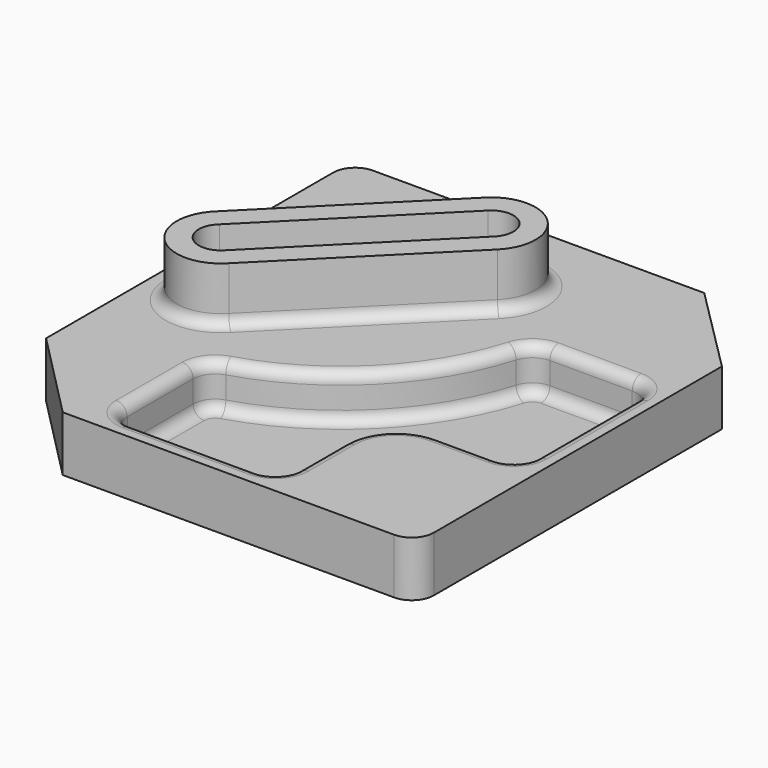
from build123d import *

# Parameters (mm, degrees)
F1_DEPTH = 25
F4_DEPTH = 25
F5_DEPTH = 5
F6_R     = 5
F7_R     = 10


with BuildPart() as f1:
    # F0 (on Top) → F1 (new body)
    with BuildSketch(Plane.XY):
        Polygon((60, 106.5), (-100, 106.5), (-100, -65.9319981933), (-60, -106.5), (100, -106.5), (100, 66.5), align=None)
        with BuildLine():
            Line((81, -37.5), (55, -37.5))
            ThreePointArc((55, -37.5), (38.0294372515, -44.5294372515), (31, -61.5))
            Line((31, -61.5), (31, -87.5))
            ThreePointArc((31, -87.5), (28.0710678119, -94.5710678119), (21, -97.5))
            Line((21, -97.5), (-36, -97.5))
            ThreePointArc((-36, -97.5), (-43.0710678119, -94.5710678119), (-46, -87.5))
            Line((-46, -87.5), (-46, -50.2086650483))
            ThreePointArc((-46, -50.2086650483), (-44.0202162123, -44.2357150312), (-38.8647736185, -40.6277949357))
            ThreePointArc((-38.8647736185, -40.6277949357), (6.8505042274, -13.3505042274), (34.1277949357, 32.3647736185))
            ThreePointArc((34.1277949357, 32.3647736185), (37.7357150312, 37.5202162123), (43.7086650483, 39.5))
            Line((43.7086650483, 39.5), (81, 39.5))
            ThreePointArc((81, 39.5), (88.0710678119, 36.5710678119), (91, 29.5))
            Line((91, 29.5), (91, -27.5))
            ThreePointArc((91, -27.5), (88.0710678119, -34.5710678119), (81, -37.5))
        make_face(mode=Mode.SUBTRACT)
    extrude(amount=F1_DEPTH)

    # F3 (on offset) → F4 (join)
    with BuildSketch(Plane(origin=(0, 0, 25), x_dir=(1, 0, 0), z_dir=(0, 0, -1))):
        with BuildLine():
            Line((12.1408432435, -49.3565721142), (-55.4461455939, 18.2180655315))
            ThreePointArc((-55.4461455939, 18.2180655315), (-84.1408590322, 18.6434121001), (-83.720692703, -10.0513776581))
            Line((-83.720692703, -10.0513776581), (-16.1434121001, -77.6408590322))
            ThreePointArc((-16.1434121001, -77.6408590322), (12.1408595897, -77.6434115426), (12.1434109852, -49.3591398528))
            ThreePointArc((12.1434109852, -49.3591398528), (12.1421271726, -49.3578559252), (12.1408432435, -49.3565721142))
        make_face()
        with BuildLine():
            ThreePointArc((-76.6428401008, -2.9748026994), (-77.0704295161, 11.57170605), (-62.5239981961, 11.1414905727))
            Line((-62.5239981961, 11.1414905727), (5.0697784915, -56.4276431028))
            ThreePointArc((5.0697784915, -56.4276431028), (5.0710717587, -70.5710638651), (-9.072349005, -70.5697863865))
            Line((-9.072349005, -70.5697863865), (-76.6428401008, -2.9748026994))
        make_face(mode=Mode.SUBTRACT)
    extrude(amount=-F4_DEPTH)

    # F0 (on Top) → F5 (join)
    with BuildSketch(Plane.XY):
        with BuildLine():
            ThreePointArc((31, -61.5), (38.0294372515, -44.5294372515), (55, -37.5))
            Line((55, -37.5), (81, -37.5))
            ThreePointArc((81, -37.5), (88.0710678119, -34.5710678119), (91, -27.5))
            Line((91, -27.5), (91, 29.5))
            ThreePointArc((91, 29.5), (88.0710678119, 36.5710678119), (81, 39.5))
            Line((81, 39.5), (43.7086650483, 39.5))
            ThreePointArc((43.7086650483, 39.5), (37.7357150312, 37.5202162123), (34.1277949357, 32.3647736185))
            ThreePointArc((34.1277949357, 32.3647736185), (6.8505042274, -13.3505042274), (-38.8647736185, -40.6277949357))
            ThreePointArc((-38.8647736185, -40.6277949357), (-44.0202162123, -44.2357150312), (-46, -50.2086650483))
            Line((-46, -50.2086650483), (-46, -87.5))
            ThreePointArc((-46, -87.5), (-43.0710678119, -94.5710678119), (-36, -97.5))
            Line((-36, -97.5), (21, -97.5))
            ThreePointArc((21, -97.5), (28.0710678119, -94.5710678119), (31, -87.5))
            Line((31, -87.5), (31, -61.5))
        make_face()
    extrude(amount=F5_DEPTH)

    # F6
    f6_edges = [f1.edges().sort_by_distance(p)[0] for p in [
        (-84.140859, -18.643412, 25),
        (-21.652651, 15.569253, 25),
        (6.850504, -13.350504, 25),
        (31, -74.5, 5),
        (38.029437, -44.529437, 5),
        (68, -37.5, 5),
        (88.071068, -34.571068, 5),
        (91, 1, 5),
        (88.071068, 36.571068, 5),
        (62.354333, 39.5, 5),
        (37.735715, 37.520216, 5),
        (6.850504, -13.350504, 5),
        (-44.020216, -44.235715, 5),
        (-46, -68.854333, 5),
        (-43.071068, -94.571068, 5),
        (-7.5, -97.5, 5),
        (28.071068, -94.571068, 5),
    ]]
    fillet(f6_edges, radius=F6_R)

    # F7
    f7_edges = [f1.edges().sort_by_distance(p)[0] for p in [
        (-100, 106.5, 12.5),
        (100, -106.5, 12.5),
    ]]
    fillet(f7_edges, radius=F7_R)


solid = f1.part
